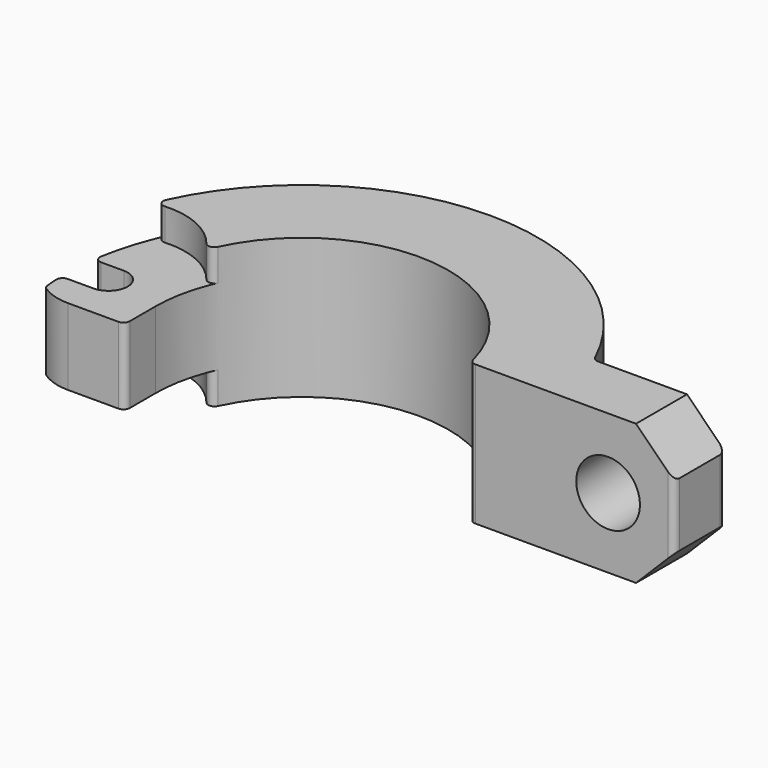
from build123d import *

# Parameters (mm, degrees)
F1_DEPTH = 5.5
F3_DEPTH = 2.5
F5_R     = 2.5
F6_DEPTH = 5
F7_SIZE  = 3
F8_R     = 0.5


# Not quite as in the source:
# - a feature names something its author has since deleted; it is built from what else it names


with BuildPart() as f1:
    # F0 (on Top) → F1 (new body)
    with BuildSketch(Plane.XY):
        with BuildLine():
            ThreePointArc((-11.5, 0), (-1.2575412829, 11.4310362576), (11.2249721603, 2.5))
            Line((11.2249721603, 2.5), (27.2249721603, 2.5))
            Line((27.2249721603, 2.5), (27.2249721603, 7.5))
            Line((27.2249721603, 7.5), (16.9115345253, 7.5))
            ThreePointArc((16.9115345253, 7.5), (-2.5986969504, 18.3165710263), (-18.3303027798, 2.5))
            Line((-18.3303027798, 2.5), (-15.9687194227, 2.5))
            ThreePointArc((-15.9687194227, 2.5), (-14.4687194227, 1), (-15.9687194227, -0.5))
            Line((-15.9687194227, -0.5), (-18.4932420089, -0.5))
            ThreePointArc((-18.4932420089, -0.5), (-18.4505725724, -1.3514332211), (-18.3687238121, -2.1999967079))
            ThreePointArc((-18.3687238121, -2.1999967079), (-17.2336330893, -2.7947323247), (-15.9687194227, -3))
            Line((-15.9687194227, -3), (-11.5, -3))
            Line((-11.5, -3), (-11.5, 0))
        make_face()
    extrude(amount=F1_DEPTH)

    # F2 (on face) → F3 (cut)
    with BuildSketch(Plane.XY.offset(5.5)):
        with BuildLine():
            Line((-15.9687194227, -3), (-11.5, -3))
            Line((-11.5, -3), (-11.5, 0))
            ThreePointArc((-11.5, 0), (-11.3184211539, 2.0355202239), (-10.7794186814, 4.0067608976))
            ThreePointArc((-10.7794186814, 4.0067608976), (-13.5146873094, 6.472401636), (-17.1751666268, 6.8748564597))
            ThreePointArc((-17.1751666268, 6.8748564597), (-17.8869905716, 4.7228771203), (-18.3303027798, 2.5))
            Line((-18.3303027798, 2.5), (-15.9687194227, 2.5))
            ThreePointArc((-15.9687194227, 2.5), (-14.4687194227, 1), (-15.9687194227, -0.5))
            Line((-15.9687194227, -0.5), (-18.4932420089, -0.5))
            ThreePointArc((-18.4932420089, -0.5), (-18.4505725724, -1.3514332211), (-18.3687238121, -2.1999967079))
            ThreePointArc((-18.3687238121, -2.1999967079), (-17.2336330893, -2.7947323247), (-15.9687194227, -3))
        make_face()
    extrude(amount=-F3_DEPTH, mode=Mode.SUBTRACT)

    # F4: F1 across plane


with BuildPart() as f1_1:
    add(f1.part)
    add(f1.part.mirror(Plane.XY))

    # F5 (on face) → F6 (cut, through all)
    with BuildSketch(Plane(origin=(0, 7.5, 0), x_dir=(-1, 0, 0), z_dir=(0, 1, 0))):
        with Locations((-22.0312805773, 0)):
            Circle(F5_R)
    extrude(amount=-F6_DEPTH, mode=Mode.SUBTRACT)

    # F7
    f7_edges = [f1_1.edges().sort_by_distance(p)[0] for p in [
        (27.224972, 5, 5.5),
        (27.224972, 5, -5.5),
    ]]
    chamfer(f7_edges, length=F7_SIZE)

    # F8
    f8_edges = [f1_1.edges().sort_by_distance(p)[0] for p in [
        (-11.5, -3, 0),
        (-10.779419, 4.006761, 4.25),
        (-10.779419, 4.006761, -4.25),
        (-17.175167, 6.874856, 4.25),
        (-17.175167, 6.874856, -4.25),
        (-18.368724, -2.199997, 0),
        (-18.493242, -0.5, 0),
        (-18.330303, 2.5, 0),
        (11.224972, 2.5, 0),
        (16.911535, 7.5, 0),
        (27.224972, 2.5, 0),
        (27.224972, 7.5, 0),
    ]]
    fillet(f8_edges, radius=F8_R)


solid = f1_1.part
